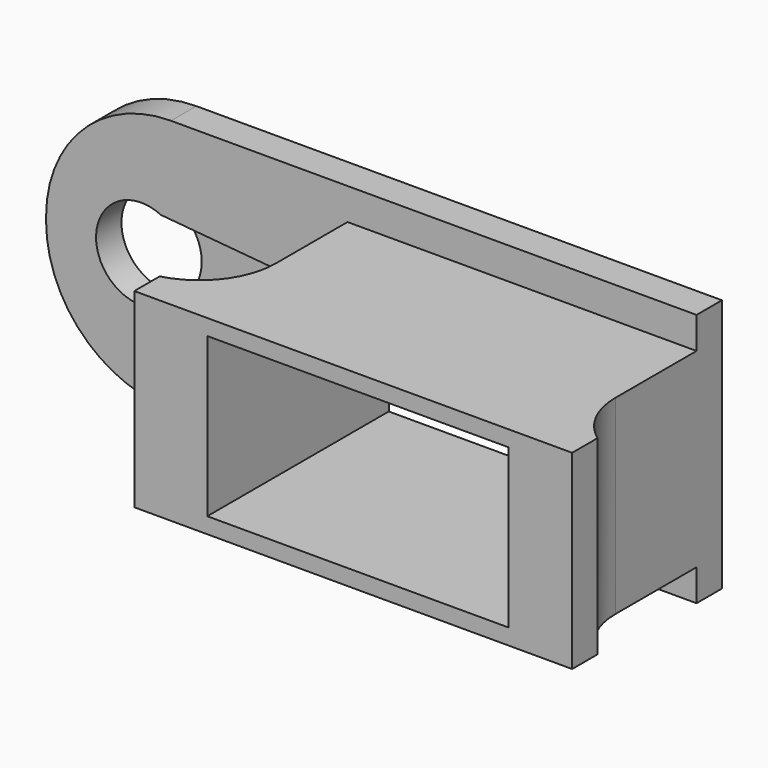
from build123d import *

# Parameters (mm, degrees)
F0_W         = 30.48
F0_H         = 20.32
F1_DEPTH     = 2.54
F2_R         = 3.6195
F4_DEPTH     = 25.4
F5_DEPTH     = 1.524
F6_DEPTH     = 21.59
F7_W         = 27.94
F7_H         = 15.24
F8_DEPTH     = 15.621
F10_DEPTH    = 25.4
F11_W        = 2.54
F11_H        = 15.24
F12_DEPTH    = 4.572
F13_W        = 2.54
F13_H        = 15.24
F14_DEPTH    = 2.54
F15_R        = 9.9953269909
F16_T1_DEPTH = 15.24


# Not quite as in the source:
# - a fillet or chamfer that OpenCascade refuses, or shapes differently, is made with other operations: its cross-section is extruded or revolved along the edge and cut away or added


with BuildPart() as f1:
    # F0 (on Front) → F1 (new body)
    with BuildSketch(Plane.XZ):
        Rectangle(F0_W, F0_H)
    extrude(amount=F1_DEPTH)

    # F2 (on face) → F4 (cut)
    with BuildSketch(Plane.XZ.offset(2.54)):
        with Locations((-7.62, 0)):
            Circle(F2_R)
    extrude(amount=-F4_DEPTH, mode=Mode.SUBTRACT)

    # F3 (on face) → F5 (cut)
    with BuildSketch(Plane.XZ.offset(2.54)):
        Polygon((7.1528805111, 2.0839335623), (-6.0890655676, 3.2650576724), (-5.9136119671, -3.1920422334), (7.1528805111, -2.0996773468), (8.7022805111, -1.0994056345), (8.7022805111, 1.1413069921), align=None)
    extrude(amount=-F5_DEPTH, mode=Mode.SUBTRACT)

    # F6 (add): a face of the model
    f6_faces = [f1.faces().sort_by_distance(p)[0] for p in [
        (15.24, -1.27, 0),
    ]]
    extrude(f6_faces, amount=F6_DEPTH)

    # F7 (on face) → F8 (join)
    with BuildSketch(Plane.XZ.offset(2.54)):
        with Locations((22.86, 0)):
            Rectangle(F7_W, F7_H)
    extrude(amount=F8_DEPTH)

    # F9 (on face) → F10 (cut)
    with BuildSketch(Plane.XZ.offset(18.161)):
        Polygon((10.16, 6.35), (10.16, -6.35), (35.56, -6.35), (35.56, 0), (35.56, 6.35), align=None)
    extrude(amount=-F10_DEPTH, mode=Mode.SUBTRACT)

    # F11 (on face) → F12 (join)
    with BuildSketch(Plane(origin=(8.89, 0, 0), x_dir=(0, -1, 0), z_dir=(-1, 0, 0))):
        with Locations((16.891, 0)):
            Rectangle(F11_W, F11_H)
    extrude(amount=F12_DEPTH)

    # F13 (on face) → F14 (join, symmetric)
    with BuildSketch(Plane.YZ.offset(36.83)):
        with Locations((-16.891, 0)):
            Rectangle(F13_W, F13_H)
    extrude(amount=F14_DEPTH, both=True)

    # F15
    f15_edges = [f1.edges().sort_by_distance(p)[0] for p in [
        (-15.24, -1.27, 10.16),
        (-15.24, -1.27, -10.16),
    ]]
    fillet(f15_edges, radius=F15_R)

    # F16: fillet of radius 6.1321024484 on 2 edges, made by hand

    # F16_s2 → F16_t1 (join)
    with BuildSketch(Plane.XY.offset(-7.62)):
        with BuildLine():
            ThreePointArc((8.89, -9.6906744787), (7.6143050963, -13.4347346007), (4.318, -15.621))
            Line((4.318, -15.621), (8.89, -15.621))
            Line((8.89, -15.621), (8.89, -9.6906744787))
        make_face()
        with BuildLine():
            ThreePointArc((36.83, -10.6511428151), (37.5017993132, -13.4418004633), (39.37, -15.621))
            Line((39.37, -15.621), (36.83, -15.621))
            Line((36.83, -15.621), (36.83, -10.6511428151))
        make_face()
    extrude(amount=F16_T1_DEPTH)


solid = f1.part
